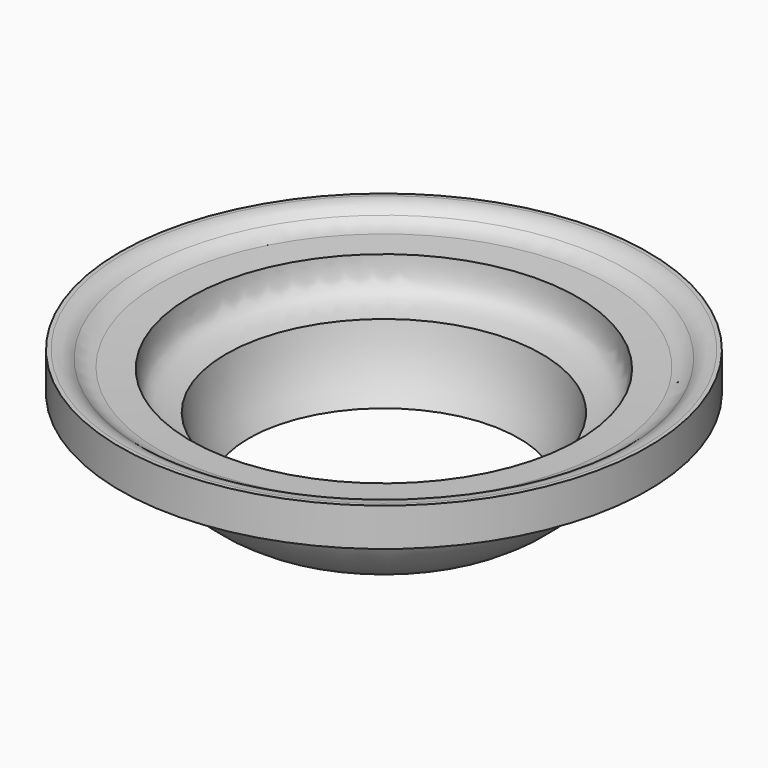
from build123d import *


# Not quite as in the source:
# - a fillet or chamfer that OpenCascade refuses, or shapes differently, is made with other operations: its cross-section is extruded or revolved along the edge and cut away or added


with BuildPart() as f1:
    # F0 (on Front) → F1 (revolve)
    with BuildSketch(Plane.XZ):
        with BuildLine():
            Line((-53.2819602912, 0), (-53.2819602912, -4.6227879951))
            Line((-53.2819602912, -4.6227879951), (-46.949992539, -4.6227879951))
            ThreePointArc((-46.949992539, -4.6227879951), (-42.687538621, -5.9264689249), (-39.883583361, -9.3914266835))
            ThreePointArc((-39.883583361, -9.3914266835), (-35.670707548, -16.3265032657), (-29.4653140008, -21.55495435))
            Line((-29.4653140008, -21.55495435), (-27.281089944, -21.55495435))
            ThreePointArc((-27.281089944, -21.55495435), (-30.3394267637, -15.0736211015), (-31.8814767831, -8.0748221676))
            add(Edge.make_bspline(
                [(-39.1281443631, -0.3240852156), (-39.0258462115, -2.415270443), (-38.815008764, -6.7252227611), (-34.2378182979, -7.6161645716), (-31.8814767831, -8.0748221676)],
                knots=[0, 0, 0, 0, 0.4851991561, 1, 1, 1, 1], degree=3))
            Line((-39.1281443631, -0.3240852156), (-45.4025, 0))
            ThreePointArc((-45.4025, 0), (-47.264175973, 0.4492875303), (-48.8369602912, 1.5420117415))
            Line((-48.8369602912, 1.5420117415), (-48.8369602912, 3.0840234831))
            Line((-48.8369602912, 3.0840234831), (-53.2819602912, 3.0840234831))
            Line((-53.2819602912, 3.0840234831), (-53.2819602912, 0))
        make_face()
    revolve(axis=Axis((0, 0, -4.7387806699), (0, 0, -1)))

    # F2: fillet of radius 5.08 on 1 edges, made by hand

    # F2_s1 → F2_t2 (revolve, cut)
    with BuildSketch(Plane.XZ):
        with BuildLine():
            ThreePointArc((-52.4823737223, 3.0840234831), (-50.5033058044, 2.6826653989), (-48.8369602912, 1.5420117415))
            Line((-48.8369602912, 1.5420117415), (-48.7640520226, 1.6127715067))
            ThreePointArc((-48.7640520226, 1.6127715067), (-48.7353602912, 2.3130176123), (-48.7353602912, 3.0840234831))
            Line((-48.7353602912, 3.0840234831), (-48.8369602912, 3.1856234831))
            Line((-48.8369602912, 3.1856234831), (-52.4823737223, 3.1856234831))
            Line((-52.4823737223, 3.1856234831), (-52.4823737223, 3.0840234831))
        make_face()
    revolve(axis=Axis((0, 0, 3.0840234831), (0, 0, -1)), mode=Mode.SUBTRACT)


solid = f1.part
